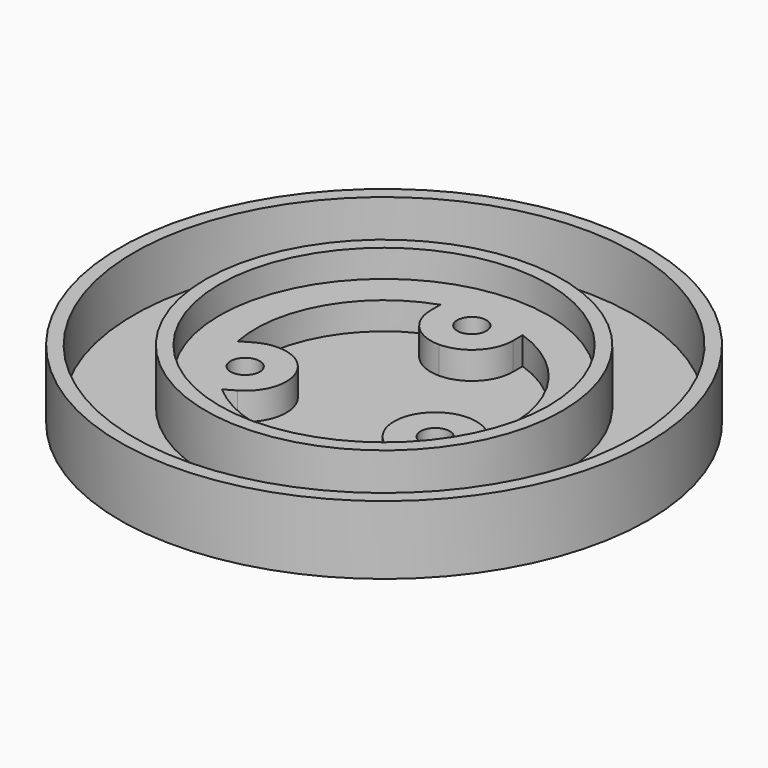
from build123d import *

# Parameters (mm, degrees)
F0_R      = 38.5
F1_DEPTH  = 2
F2_R      = 38.5
F2_R_2    = 36.5
F3_DEPTH  = 8
F4_R      = 26
F4_R_2    = 24
F5_DEPTH  = 8
F6_R      = 24
F6_R_2    = 18.75
F7_DEPTH  = 4
F8_R      = 2.125
F9_DEPTH  = 12.5
F10_R     = 2.125
F11_DEPTH = 4
F12_R     = 5.99999


# Not quite as in the source:
# - a fillet or chamfer is up to 0.001 mm smaller than in the source, because OpenCascade refuses the exact size


with BuildPart() as f1:
    # F0 (on Top) → F1 (new body)
    with BuildSketch(Plane.XY):
        Circle(F0_R)
    extrude(amount=F1_DEPTH)

    # F2 (on face) → F3 (join)
    with BuildSketch(Plane.XY.offset(2)):
        Circle(F2_R)
        Circle(F2_R_2, mode=Mode.SUBTRACT)
    extrude(amount=F3_DEPTH)

    # F4 (on face) → F5 (join)
    with BuildSketch(Plane.XY.offset(2)):
        Circle(F4_R)
        Circle(F4_R_2, mode=Mode.SUBTRACT)
    extrude(amount=F5_DEPTH)

    # F6 (on face) → F7 (join)
    with BuildSketch(Plane.XY.offset(2)):
        Circle(F6_R)
        Circle(F6_R_2, mode=Mode.SUBTRACT)
    extrude(amount=F7_DEPTH)

    # F8 (on face) → F9 (cut, symmetric)
    with BuildSketch(Plane.XY.offset(2)):
        with Locations((0, 16)):
            Circle(F8_R)
        with Locations((-13.8564064606, -8)):
            Circle(F8_R)
        with Locations((13.8564064606, -8)):
            Circle(F8_R)
    extrude(amount=F9_DEPTH, both=True, mode=Mode.SUBTRACT)

    # F10 (on face) → F11 (join)
    with BuildSketch(Plane.XY.offset(2)):
        with BuildLine():
            Line((6, 16), (6, 17.7640789235))
            ThreePointArc((6, 17.7640789235), (0, 18.75), (-6, 17.7640789235))
            Line((-6, 17.7640789235), (-6, 16))
            Line((-6, 16), (-6, 10))
            Line((-6, 10), (0, 10))
            Line((0, 10), (6, 10))
            Line((6, 10), (6, 16))
        make_face()
        with Locations((0, 16)):
            Circle(F10_R, mode=Mode.SUBTRACT)
        with BuildLine():
            Line((-16.8564064606, -2.8038475773), (-18.3841436226, -3.685887039))
            ThreePointArc((-18.3841436226, -3.685887039), (-16.237976321, -9.375), (-12.3841436226, -14.0781918845))
            Line((-12.3841436226, -14.0781918845), (-10.8564064606, -13.1961524227))
            Line((-10.8564064606, -13.1961524227), (-5.6602540378, -10.1961524227))
            Line((-5.6602540378, -10.1961524227), (-8.6602540378, -5))
            Line((-8.6602540378, -5), (-11.6602540378, 0.1961524227))
            Line((-11.6602540378, 0.1961524227), (-16.8564064606, -2.8038475773))
        make_face()
        with Locations((-13.8564064606, -8)):
            Circle(F10_R, mode=Mode.SUBTRACT)
        with BuildLine():
            ThreePointArc((12.3841436226, -14.0781918845), (16.237976321, -9.375), (18.3841436226, -3.685887039))
            Line((18.3841436226, -3.685887039), (16.8564064606, -2.8038475773))
            Line((16.8564064606, -2.8038475773), (11.6602540378, 0.1961524227))
            Line((11.6602540378, 0.1961524227), (8.6602540378, -5))
            Line((8.6602540378, -5), (5.6602540378, -10.1961524227))
            Line((5.6602540378, -10.1961524227), (10.8564064606, -13.1961524227))
            Line((10.8564064606, -13.1961524227), (12.3841436226, -14.0781918845))
        make_face()
        with Locations((13.8564064606, -8)):
            Circle(F10_R, mode=Mode.SUBTRACT)
    extrude(amount=F11_DEPTH)

    # F12 (radius 6 in the source; OpenCascade refuses exactly that, so slightly less here)
    f12_edges = [f1.edges().sort_by_distance(p)[0] for p in [
        (-6, 10, 4),
        (6, 10, 4),
        (11.660254, 0.196152, 4),
        (5.660254, -10.196152, 4),
        (-5.660254, -10.196152, 4),
        (-11.660254, 0.196152, 4),
    ]]
    fillet(f12_edges, radius=F12_R)


solid = f1.part
